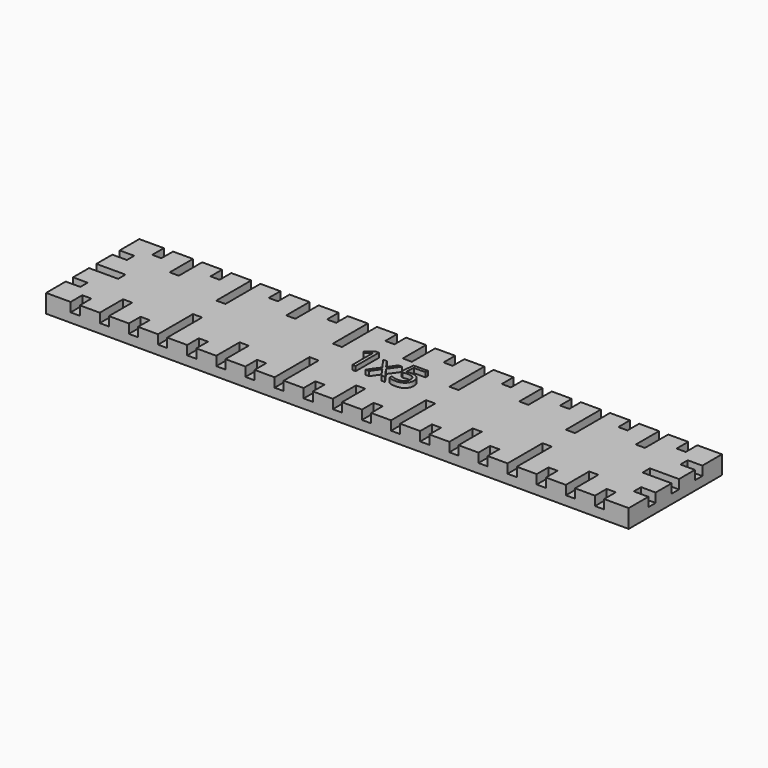
from build123d import *

# Parameters (mm, degrees)
F0_W         = 127
F0_H         = 25.4
F1_DEPTH     = 4
F2_W         = 2
F2_H         = 12.7
F2_H_2       = 6.35
F2_W_2       = 12.7
F2_H_3       = 2
F2_W_3       = 6.35
F2_H_4       = 19.05
F2_W_4       = 1.9981167428
F2_W_5       = 0.0018831447
F2_H_5       = 6.3500001945
F2_W_6       = 0.0018832572
F2_H_6       = 6.3500000358
F3_DEPTH     = 2
F4_TEXT_SIZE = 8.8296504044
F5_DEPTH     = 1


# Not quite as in the source:
# - ends of sketch curves that miss each other by under 0.0002 mm in the source are joined
# - Text() gives the source's letters only with a copy of the font that has no kerning and outlines rounded to 1/6400 em; it was checked with that copy


with BuildPart() as f1:
    # F0 (on Top) → F1 (new body)
    with BuildSketch(Plane.XY):
        Rectangle(F0_W, F0_H)
    extrude(amount=F1_DEPTH)

    # F2 (on face) → F3 (cut)
    with BuildSketch(Plane.XY.offset(4)):
        with Locations((0, -12.7)):
            Rectangle(F2_W, F2_H)
        with Locations((6.35, -12.7)):
            Rectangle(F2_W, F2_H_2)
        with Locations((-6.35, -12.7)):
            Rectangle(F2_W, F2_H_2)
        with Locations((-63.5, 0)):
            Rectangle(F2_W_2, F2_H_3)
        with Locations((-63.5, 6.35)):
            Rectangle(F2_W_3, F2_H_3)
        with Locations((-63.5, -6.35)):
            Rectangle(F2_W_3, F2_H_3)
        with Locations((0, 12.7)):
            Rectangle(F2_W, F2_H)
        with Locations((-6.35, 12.7)):
            Rectangle(F2_W, F2_H_2)
        with Locations((6.35, 12.7)):
            Rectangle(F2_W, F2_H_2)
        with Locations((63.5, 0)):
            Rectangle(F2_W_2, F2_H_3)
        with Locations((63.5, -6.35)):
            Rectangle(F2_W_3, F2_H_3)
        with Locations((63.5, 6.35)):
            Rectangle(F2_W_3, F2_H_3)
        with Locations((-12.7, 12.7000001177)):
            Rectangle(F2_W, F2_H_4)
        with Locations((-19.05, 12.7000001177)):
            Rectangle(F2_W, F2_H_2)
        with Locations((-12.7, -12.7000005066)):
            Rectangle(F2_W, F2_H_4)
        with Locations((-19.05, -12.7000005066)):
            Rectangle(F2_W, F2_H_2)
        with Locations((12.700000225, -12.7)):
            Rectangle(F2_W, F2_H_4)
        with Locations((19.050000225, -12.7)):
            Rectangle(F2_W, F2_H_2)
        with Locations((12.700000225, 12.7)):
            Rectangle(F2_W, F2_H_4)
        with Locations((19.050000225, 12.7)):
            Rectangle(F2_W, F2_H_2)
        with Locations((25.4000000715, 12.7)):
            Rectangle(F2_W, F2_H)
        with Locations((31.7509417001, 12.7)):
            Rectangle(F2_W_4, F2_H_2)
        with Locations((32.7509416439, 12.7000000972)):
            Rectangle(F2_W_5, F2_H_5)
        with Locations((30.7509417001, 12.7000000972)):
            Rectangle(F2_W_6, F2_H_5)
        with Locations((25.4000000715, -12.7)):
            Rectangle(F2_W, F2_H)
        with Locations((31.7509417001, -12.7)):
            Rectangle(F2_W_4, F2_H_2)
        with Locations((32.7509416439, -12.6999999821)):
            Rectangle(F2_W_5, F2_H_6)
        with Locations((30.7509417001, -12.6999999821)):
            Rectangle(F2_W_6, F2_H_6)
        with Locations((-25.4000000715, -12.7000005066)):
            Rectangle(F2_W, F2_H)
        with Locations((-31.7500000715, -12.7000005066)):
            Rectangle(F2_W, F2_H_2)
        with Locations((-25.4, 12.7000005066)):
            Rectangle(F2_W, F2_H)
        with Locations((-31.75, 12.7000005066)):
            Rectangle(F2_W, F2_H_2)
        with Locations((38.1018834412, 12.7000001945)):
            Rectangle(F2_W, F2_H_4)
        with Locations((44.4518834412, 12.7000001945)):
            Rectangle(F2_W, F2_H_2)
        with Locations((50.8018832877, 12.7000001945)):
            Rectangle(F2_W, F2_H)
        with Locations((57.1518832877, 12.7000001945)):
            Rectangle(F2_W, F2_H_2)
        with Locations((38.1018834412, -12.6999999642)):
            Rectangle(F2_W, F2_H_4)
        with Locations((44.4518834412, -12.6999999642)):
            Rectangle(F2_W, F2_H_2)
        with Locations((50.8018832877, -12.6999999642)):
            Rectangle(F2_W, F2_H)
        with Locations((57.1518832877, -12.6999999642)):
            Rectangle(F2_W, F2_H_2)
        with Locations((-38.099968642, -12.7000004273)):
            Rectangle(F2_W, F2_H_4)
        with Locations((-44.449968642, -12.7000004273)):
            Rectangle(F2_W, F2_H_2)
        with Locations((-50.7999684885, -12.7000004273)):
            Rectangle(F2_W, F2_H)
        with Locations((-57.1499684885, -12.7000004273)):
            Rectangle(F2_W, F2_H_2)
        with Locations((-38.099968642, 12.6999999642)):
            Rectangle(F2_W, F2_H_4)
        with Locations((-44.449968642, 12.6999999642)):
            Rectangle(F2_W, F2_H_2)
        with Locations((-50.7999684885, 12.6999999642)):
            Rectangle(F2_W, F2_H)
        with Locations((-57.1499684885, 12.6999999642)):
            Rectangle(F2_W, F2_H_2)
    extrude(amount=-F3_DEPTH, mode=Mode.SUBTRACT)

    # F4 (on face) → F5 (join)
    with BuildSketch(Plane.XY.offset(4)):
        with Locations((-7.3934525809, -2.3339281324)):
            Text('1x5', F4_TEXT_SIZE, font='Open Sans', text_align=(TextAlign.LEFT, TextAlign.BOTTOM))
    extrude(amount=F5_DEPTH)


solid = f1.part
